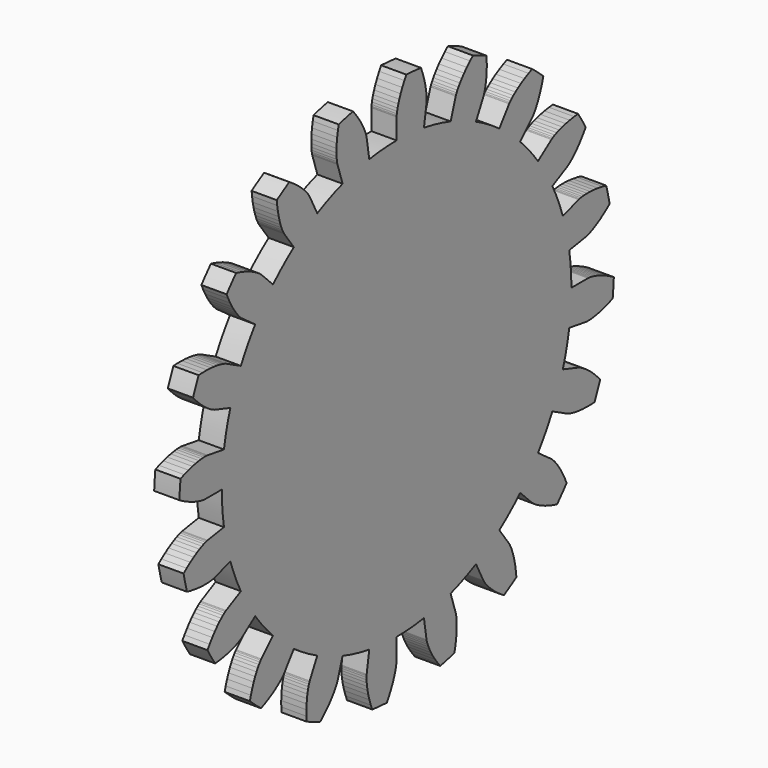
from build123d import *

# Parameters (mm, degrees)
F2_DEPTH = 5.08


# Not quite as in the source:
# - a variable given as a bare number and used for a length is read in inches; the dataset says mm whatever the document's units were


with BuildPart() as f2:
    # F1 (on Right) → F2 (new body)
    with BuildSketch(Plane.YZ):
        with BuildLine():
            ThreePointArc((43.4993825677, -6.8896253625), (43.9058422643, -3.4554647258), (44.0416078431, 0))
            ThreePointArc((44.0416078431, 0), (43.9058422643, 3.4554647258), (43.4993825677, 6.8896253625))
            ThreePointArc((43.4993825677, 6.8896253625), (42.8247347126, 10.2813091677), (41.8860581273, 13.6096052831))
            ThreePointArc((41.8860581273, 13.6096052831), (40.6891400652, 16.8539936563), (39.241359924, 19.994471554))
            ThreePointArc((39.241359924, 19.994471554), (37.5516437498, 23.0116768858), (35.6304092047, 25.8870075774))
            ThreePointArc((35.6304092047, 25.8870075774), (33.4895013385, 28.602736259), (31.1421195602, 31.1421195602))
            ThreePointArc((31.1421195602, 31.1421195602), (28.602736259, 33.4895013385), (25.8870075774, 35.6304092047))
            ThreePointArc((25.8870075774, 35.6304092047), (23.0116768858, 37.5516437498), (19.994471554, 39.241359924))
            ThreePointArc((19.994471554, 39.241359924), (16.8539936563, 40.6891400652), (13.6096052831, 41.8860581273))
            ThreePointArc((13.6096052831, 41.8860581273), (10.2813091677, 42.8247347126), (6.8896253625, 43.4993825677))
            ThreePointArc((6.8896253625, 43.4993825677), (3.4554647258, 43.9058422643), (0, 44.0416078431))
            ThreePointArc((0, 44.0416078431), (-3.4554647258, 43.9058422643), (-6.8896253625, 43.4993825677))
            ThreePointArc((-6.8896253625, 43.4993825677), (-10.2813091677, 42.8247347126), (-13.6096052831, 41.8860581273))
            ThreePointArc((-13.6096052831, 41.8860581273), (-16.8539936563, 40.6891400652), (-19.994471554, 39.241359924))
            ThreePointArc((-19.994471554, 39.241359924), (-23.0116768858, 37.5516437498), (-25.8870075774, 35.6304092047))
            ThreePointArc((-25.8870075774, 35.6304092047), (-28.602736259, 33.4895013385), (-31.1421195602, 31.1421195602))
            ThreePointArc((-31.1421195602, 31.1421195602), (-33.4895013385, 28.602736259), (-35.6304092047, 25.8870075774))
            ThreePointArc((-35.6304092047, 25.8870075774), (-37.5516437498, 23.0116768858), (-39.241359924, 19.994471554))
            ThreePointArc((-39.241359924, 19.994471554), (-40.6891400652, 16.8539936563), (-41.8860581273, 13.6096052831))
            ThreePointArc((-41.8860581273, 13.6096052831), (-42.8247347126, 10.2813091677), (-43.4993825677, 6.8896253625))
            ThreePointArc((-43.4993825677, 6.8896253625), (-43.9058422643, 3.4554647258), (-44.0416078431, 0))
            ThreePointArc((-44.0416078431, 0), (-43.9058422643, -3.4554647258), (-43.4993825677, -6.8896253625))
            ThreePointArc((-43.4993825677, -6.8896253625), (-42.8247347126, -10.2813091677), (-41.8860581273, -13.6096052831))
            ThreePointArc((-41.8860581273, -13.6096052831), (-40.6891400652, -16.8539936563), (-39.241359924, -19.994471554))
            ThreePointArc((-39.241359924, -19.994471554), (-37.5516437498, -23.0116768858), (-35.6304092047, -25.8870075774))
            ThreePointArc((-35.6304092047, -25.8870075774), (-33.4895013385, -28.602736259), (-31.1421195602, -31.1421195602))
            ThreePointArc((-31.1421195602, -31.1421195602), (-28.602736259, -33.4895013385), (-25.8870075774, -35.6304092047))
            ThreePointArc((-25.8870075774, -35.6304092047), (-23.0116768858, -37.5516437498), (-19.994471554, -39.241359924))
            ThreePointArc((-19.994471554, -39.241359924), (-16.8539936563, -40.6891400652), (-13.6096052831, -41.8860581273))
            ThreePointArc((-13.6096052831, -41.8860581273), (-10.2813091677, -42.8247347126), (-6.8896253625, -43.4993825677))
            ThreePointArc((-6.8896253625, -43.4993825677), (-3.4554647258, -43.9058422643), (0, -44.0416078431))
            ThreePointArc((0, -44.0416078431), (3.4554647258, -43.9058422643), (6.8896253625, -43.4993825677))
            ThreePointArc((6.8896253625, -43.4993825677), (10.2813091677, -42.8247347126), (13.6096052831, -41.8860581273))
            ThreePointArc((13.6096052831, -41.8860581273), (16.8539936563, -40.6891400652), (19.994471554, -39.241359924))
            ThreePointArc((19.994471554, -39.241359924), (23.0116768858, -37.5516437498), (25.8870075774, -35.6304092047))
            ThreePointArc((25.8870075774, -35.6304092047), (28.602736259, -33.4895013385), (31.1421195602, -31.1421195602))
            ThreePointArc((31.1421195602, -31.1421195602), (33.4895013385, -28.602736259), (35.6304092047, -25.8870075774))
            ThreePointArc((35.6304092047, -25.8870075774), (37.5516437498, -23.0116768858), (39.241359924, -19.994471554))
            ThreePointArc((39.241359924, -19.994471554), (40.6891400652, -16.8539936563), (41.8860581273, -13.6096052831))
            ThreePointArc((41.8860581273, -13.6096052831), (42.8247347126, -10.2813091677), (43.4993825677, -6.8896253625))
        make_face()
        with BuildLine():
            Line((-45.8576143172, -14.9000421139), (-41.8860581273, -13.6096052831))
            ThreePointArc((-41.8860581273, -13.6096052831), (-42.8247347126, -10.2813091677), (-43.4993825677, -6.8896253625))
            Line((-43.4993825677, -6.8896253625), (-47.6239111058, -7.5428865066))
            Line((-47.6239111058, -7.5428865066), (-47.6830895909, -7.554293021))
            Line((-47.6830895909, -7.554293021), (-47.8589239222, -7.5963654027))
            Line((-47.8589239222, -7.5963654027), (-48.1482035174, -7.6807235949))
            Line((-48.1482035174, -7.6807235949), (-48.5468516924, -7.8187286981))
            Line((-48.5468516924, -7.8187286981), (-49.0499442332, -8.0214256496))
            Line((-49.0499442332, -8.0214256496), (-49.6517315213, -8.2994871485))
            Line((-49.6517315213, -8.2994871485), (-50.345664133, -8.6631590363))
            Line((-50.345664133, -8.6631590363), (-51.1244218199, -9.1222073416))
            Line((-51.1244218199, -9.1222073416), (-51.9799457672, -9.6858671883))
            Line((-51.9799457672, -9.6858671883), (-52.9034740144, -10.3627937613))
            Line((-52.9034740144, -10.3627937613), (-53.6713125986, -10.9868664465))
            ThreePointArc((-53.6713125986, -10.9868664465), (-53.2706187763, -12.7891440512), (-52.8094226758, -14.5768963441))
            Line((-52.8094226758, -14.5768963441), (-51.8419504174, -14.7843577556))
            Line((-51.8419504174, -14.7843577556), (-50.7117624908, -14.9682306981))
            Line((-50.7117624908, -14.9682306981), (-49.6935888566, -15.0820555545))
            Line((-49.6935888566, -15.0820555545), (-48.7913071073, -15.1375219981))
            Line((-48.7913071073, -15.1375219981), (-48.0079050409, -15.1465172096))
            Line((-48.0079050409, -15.1465172096), (-47.3454713621, -15.1210661075))
            Line((-47.3454713621, -15.1210661075), (-46.8051901357, -15.0732711798))
            Line((-46.8051901357, -15.0732711798), (-46.3873390052, -15.0152521429))
            Line((-46.3873390052, -15.0152521429), (-46.0912911807, -14.9590856545))
            Line((-46.0912911807, -14.9590856545), (-45.9155211827, -14.9167453051))
            Line((-45.9155211827, -14.9167453051), (-45.8576143172, -14.9000421139))
        make_face()
        with BuildLine():
            Line((-39.008816688, -28.341564291), (-35.6304092047, -25.8870075774))
            ThreePointArc((-35.6304092047, -25.8870075774), (-37.5516437498, -23.0116768858), (-39.241359924, -19.994471554))
            Line((-39.241359924, -19.994471554), (-42.9621508715, -21.890309234))
            Line((-42.9621508715, -21.890309234), (-43.0149081485, -21.9194446315))
            Line((-43.0149081485, -21.9194446315), (-43.1691354541, -22.0137936409))
            Line((-43.1691354541, -22.0137936409), (-43.4181885832, -22.1834153603))
            Line((-43.4181885832, -22.1834153603), (-43.7546796056, -22.4378550738))
            Line((-43.7546796056, -22.4378550738), (-44.170512242, -22.7860954753))
            Line((-44.170512242, -22.7860954753), (-44.6569202352, -23.2365101747))
            Line((-44.6569202352, -23.2365101747), (-45.2045085737, -23.7968196633))
            Line((-45.2045085737, -23.7968196633), (-45.8032974188, -24.4740499052))
            Line((-45.8032974188, -24.4740499052), (-46.4427685721, -25.2744937142))
            Line((-46.4427685721, -25.2744937142), (-47.1119143146, -26.2036750656))
            Line((-47.1119143146, -26.2036750656), (-47.6493231381, -27.034478631))
            ThreePointArc((-47.6493231381, -27.034478631), (-46.7113062589, -28.6247252905), (-45.720236862, -30.1824613253))
            Line((-45.720236862, -30.1824613253), (-44.7360069646, -30.0808034832))
            Line((-44.7360069646, -30.0808034832), (-43.6043145082, -29.9064297672))
            Line((-43.6043145082, -29.9064297672), (-42.6008000237, -29.7000506824))
            Line((-42.6008000237, -29.7000506824), (-41.7255390128, -29.4739820107))
            Line((-41.7255390128, -29.4739820107), (-40.9776996994, -29.2404524133))
            Line((-40.9776996994, -29.2404524133), (-40.3555526557, -29.0115437125))
            Line((-40.3555526557, -29.0115437125), (-39.8564841196, -28.7991319543))
            Line((-39.8564841196, -28.7991319543), (-39.4770129475, -28.6148294707))
            Line((-39.4770129475, -28.6148294707), (-39.2128111343, -28.469928157))
            Line((-39.2128111343, -28.469928157), (-39.0587278198, -28.3753441754))
            Line((-39.0587278198, -28.3753441754), (-39.008816688, -28.341564291))
        make_face()
        with BuildLine():
            Line((-28.341564291, -39.008816688), (-25.8870075774, -35.6304092047))
            ThreePointArc((-25.8870075774, -35.6304092047), (-28.602736259, -33.4895013385), (-31.1421195602, -31.1421195602))
            Line((-31.1421195602, -31.1421195602), (-34.0949559749, -34.0949559749))
            Line((-34.0949559749, -34.0949559749), (-34.1361277941, -34.1389682797))
            Line((-34.1361277941, -34.1389682797), (-34.2536512308, -34.2763583784))
            Line((-34.2536512308, -34.2763583784), (-34.4380988382, -34.5146398693))
            Line((-34.4380988382, -34.5146398693), (-34.6794946222, -34.8606078612))
            Line((-34.6794946222, -34.8606078612), (-34.9673627586, -35.3203035157))
            Line((-34.9673627586, -35.3203035157), (-35.2907784534, -35.8989816867))
            Line((-35.2907784534, -35.8989816867), (-35.6384207569, -36.6010817796))
            Line((-35.6384207569, -36.6010817796), (-35.9986271361, -37.4302019433))
            Line((-35.9986271361, -37.4302019433), (-36.3594496034, -38.3890766975))
            Line((-36.3594496034, -38.3890766975), (-36.7087121936, -39.4795580828))
            Line((-36.7087121936, -39.4795580828), (-36.9630859365, -40.4357676868))
            ThreePointArc((-36.9630859365, -40.4357676868), (-35.5795656281, -41.6583189782), (-34.1556357126, -42.8335566985))
            Line((-34.1556357126, -42.8335566985), (-33.2509914559, -42.4327305806))
            Line((-33.2509914559, -42.4327305806), (-32.2285724125, -41.9171791203))
            Line((-32.2285724125, -41.9171791203), (-31.3379480673, -41.4107979171))
            Line((-31.3379480673, -41.4107979171), (-30.5753844409, -40.9253233069))
            Line((-30.5753844409, -40.9253233069), (-29.936311603, -40.4721284046))
            Line((-29.936311603, -40.4721284046), (-29.4153512817, -40.0621692835))
            Line((-29.4153512817, -40.0621692835), (-29.0063477414, -39.7059330378))
            Line((-29.0063477414, -39.7059330378), (-28.70240181, -39.4133879188))
            Line((-28.70240181, -39.4133879188), (-28.4959079224, -39.1939357299))
            Line((-28.4959079224, -39.1939357299), (-28.3785940398, -39.0563666551))
            Line((-28.3785940398, -39.0563666551), (-28.341564291, -39.008816688))
        make_face()
        with BuildLine():
            Line((-14.9000421139, -45.8576143172), (-13.6096052831, -41.8860581273))
            ThreePointArc((-13.6096052831, -41.8860581273), (-16.8539936563, -40.6891400652), (-19.994471554, -39.241359924))
            Line((-19.994471554, -39.241359924), (-21.890309234, -42.9621508715))
            Line((-21.890309234, -42.9621508715), (-21.9158654108, -43.0167318526))
            Line((-21.9158654108, -43.0167318526), (-21.9851809658, -43.1837143403))
            Line((-21.9851809658, -43.1837143403), (-22.0869680345, -43.4673309502))
            Line((-22.0869680345, -43.4673309502), (-22.2096390789, -43.8709614629))
            Line((-22.2096390789, -43.8709614629), (-22.3413641764, -44.397114157))
            Line((-22.3413641764, -44.397114157), (-22.4701293913, -45.0474107484))
            Line((-22.4701293913, -45.0474107484), (-22.5837960089, -45.8225749965))
            Line((-22.5837960089, -45.8225749965), (-22.6701604121, -46.7224250236))
            Line((-22.6701604121, -46.7224250236), (-22.7170143763, -47.7458693813))
            Line((-22.7170143763, -47.7458693813), (-22.7122055586, -48.8909068846))
            Line((-22.7122055586, -48.8909068846), (-22.6586443465, -49.8789220689))
            ThreePointArc((-22.6586443465, -49.8789220689), (-20.9650492162, -50.6141061537), (-19.2476429633, -51.2918051031))
            Line((-19.2476429633, -51.2918051031), (-18.5111372303, -50.6310463626))
            Line((-18.5111372303, -50.6310463626), (-17.6980730994, -49.824782927))
            Line((-17.6980730994, -49.824782927), (-17.0075194097, -49.0679677257))
            Line((-17.0075194097, -49.0679677257), (-16.4322982086, -48.3706088143))
            Line((-16.4322982086, -48.3706088143), (-15.9645487484, -47.7421104818))
            Line((-15.9645487484, -47.7421104818), (-15.5957703755, -47.1912305956))
            Line((-15.5957703755, -47.1912305956), (-15.3168679472, -46.726040748))
            Line((-15.3168679472, -46.726040748), (-15.1181996019, -46.3538893481))
            Line((-15.1181996019, -46.3538893481), (-14.9896267004, -46.0813677933))
            Line((-14.9896267004, -46.0813677933), (-14.9205657499, -45.914279845))
            Line((-14.9205657499, -45.914279845), (-14.9000421139, -45.8576143172))
        make_face()
        with BuildLine():
            Line((0, -48.2175491482), (0, -44.0416078431))
            ThreePointArc((0, -44.0416078431), (-3.4554647258, -43.9058422643), (-6.8896253625, -43.4993825677))
            Line((-6.8896253625, -43.4993825677), (-7.5428865066, -47.6239111058))
            Line((-7.5428865066, -47.6239111058), (-7.5503254243, -47.6837179965))
            Line((-7.5503254243, -47.6837179965), (-7.564648008, -47.863947464))
            Line((-7.564648008, -47.863947464), (-7.5738109107, -48.1651368231))
            Line((-7.5738109107, -48.1651368231), (-7.5657493189, -48.5869196898))
            Line((-7.5657493189, -48.5869196898), (-7.5284372071, -49.1280259317))
            Line((-7.5284372071, -49.1280259317), (-7.4499475057, -49.7862853821))
            Line((-7.4499475057, -49.7862853821), (-7.318511957, -50.5586353081))
            Line((-7.318511957, -50.5586353081), (-7.1225804347, -51.4411316084))
            Line((-7.1225804347, -51.4411316084), (-6.8508795033, -52.428963705))
            Line((-6.8508795033, -52.428963705), (-6.4924699982, -53.5164730775))
            Line((-6.4924699982, -53.5164730775), (-6.1362167757, -54.4395800319))
            ThreePointArc((-6.1362167757, -54.4395800319), (-4.298327715, -54.6154319696), (-2.4555568145, -54.7292542531))
            Line((-2.4555568145, -54.7292542531), (-1.9592839178, -53.8732425593))
            Line((-1.9592839178, -53.8732425593), (-1.4351630815, -52.8551898311))
            Line((-1.4351630815, -52.8551898311), (-1.0122762539, -51.9220229766))
            Line((-1.0122762539, -51.9220229766), (-0.6807041371, -51.0810421131))
            Line((-0.6807041371, -51.0810421131), (-0.4300646306, -50.3387621461))
            Line((-0.4300646306, -50.3387621461), (-0.2495668027, -49.7008854563))
            Line((-0.2495668027, -49.7008854563), (-0.1280663995, -49.1722780304))
            Line((-0.1280663995, -49.1722780304), (-0.0541226821, -48.7569491214))
            Line((-0.0541226821, -48.7569491214), (-0.016056378, -48.4580345094))
            Line((-0.016056378, -48.4580345094), (-0.0020085267, -48.27778342))
            Line((-0.0020085267, -48.27778342), (0, -48.2175491482))
        make_face()
        with BuildLine():
            Line((14.9000421139, -45.8576143172), (13.6096052831, -41.8860581273))
            ThreePointArc((13.6096052831, -41.8860581273), (10.2813091677, -42.8247347126), (6.8896253625, -43.4993825677))
            Line((6.8896253625, -43.4993825677), (7.5428865066, -47.6239111058))
            Line((7.5428865066, -47.6239111058), (7.554293021, -47.6830895909))
            Line((7.554293021, -47.6830895909), (7.5963654027, -47.8589239222))
            Line((7.5963654027, -47.8589239222), (7.6807235949, -48.1482035174))
            Line((7.6807235949, -48.1482035174), (7.8187286981, -48.5468516924))
            Line((7.8187286981, -48.5468516924), (8.0214256496, -49.0499442332))
            Line((8.0214256496, -49.0499442332), (8.2994871485, -49.6517315213))
            Line((8.2994871485, -49.6517315213), (8.6631590363, -50.345664133))
            Line((8.6631590363, -50.345664133), (9.1222073416, -51.1244218199))
            Line((9.1222073416, -51.1244218199), (9.6858671883, -51.9799457672))
            Line((9.6858671883, -51.9799457672), (10.3627937613, -52.9034740144))
            Line((10.3627937613, -52.9034740144), (10.9868664465, -53.6713125986))
            ThreePointArc((10.9868664465, -53.6713125986), (12.7891440512, -53.2706187763), (14.5768963441, -52.8094226758))
            Line((14.5768963441, -52.8094226758), (14.7843577556, -51.8419504174))
            Line((14.7843577556, -51.8419504174), (14.9682306981, -50.7117624908))
            Line((14.9682306981, -50.7117624908), (15.0820555545, -49.6935888566))
            Line((15.0820555545, -49.6935888566), (15.1375219981, -48.7913071073))
            Line((15.1375219981, -48.7913071073), (15.1465172096, -48.0079050409))
            Line((15.1465172096, -48.0079050409), (15.1210661075, -47.3454713621))
            Line((15.1210661075, -47.3454713621), (15.0732711798, -46.8051901357))
            Line((15.0732711798, -46.8051901357), (15.0152521429, -46.3873390052))
            Line((15.0152521429, -46.3873390052), (14.9590856545, -46.0912911807))
            Line((14.9590856545, -46.0912911807), (14.9167453051, -45.9155211827))
            Line((14.9167453051, -45.9155211827), (14.9000421139, -45.8576143172))
        make_face()
        with BuildLine():
            Line((28.341564291, -39.008816688), (25.8870075774, -35.6304092047))
            ThreePointArc((25.8870075774, -35.6304092047), (23.0116768858, -37.5516437498), (19.994471554, -39.241359924))
            Line((19.994471554, -39.241359924), (21.890309234, -42.9621508715))
            Line((21.890309234, -42.9621508715), (21.9194446315, -43.0149081485))
            Line((21.9194446315, -43.0149081485), (22.0137936409, -43.1691354541))
            Line((22.0137936409, -43.1691354541), (22.1834153603, -43.4181885832))
            Line((22.1834153603, -43.4181885832), (22.4378550738, -43.7546796056))
            Line((22.4378550738, -43.7546796056), (22.7860954753, -44.170512242))
            Line((22.7860954753, -44.170512242), (23.2365101747, -44.6569202352))
            Line((23.2365101747, -44.6569202352), (23.7968196633, -45.2045085737))
            Line((23.7968196633, -45.2045085737), (24.4740499052, -45.8032974188))
            Line((24.4740499052, -45.8032974188), (25.2744937142, -46.4427685721))
            Line((25.2744937142, -46.4427685721), (26.2036750656, -47.1119143146))
            Line((26.2036750656, -47.1119143146), (27.034478631, -47.6493231381))
            ThreePointArc((27.034478631, -47.6493231381), (28.6247252905, -46.7113062589), (30.1824613253, -45.720236862))
            Line((30.1824613253, -45.720236862), (30.0808034832, -44.7360069646))
            Line((30.0808034832, -44.7360069646), (29.9064297672, -43.6043145082))
            Line((29.9064297672, -43.6043145082), (29.7000506824, -42.6008000237))
            Line((29.7000506824, -42.6008000237), (29.4739820107, -41.7255390128))
            Line((29.4739820107, -41.7255390128), (29.2404524133, -40.9776996994))
            Line((29.2404524133, -40.9776996994), (29.0115437125, -40.3555526557))
            Line((29.0115437125, -40.3555526557), (28.7991319543, -39.8564841196))
            Line((28.7991319543, -39.8564841196), (28.6148294707, -39.4770129475))
            Line((28.6148294707, -39.4770129475), (28.469928157, -39.2128111343))
            Line((28.469928157, -39.2128111343), (28.3753441754, -39.0587278198))
            Line((28.3753441754, -39.0587278198), (28.341564291, -39.008816688))
        make_face()
        with BuildLine():
            Line((39.008816688, -28.341564291), (35.6304092047, -25.8870075774))
            ThreePointArc((35.6304092047, -25.8870075774), (33.4895013385, -28.602736259), (31.1421195602, -31.1421195602))
            Line((31.1421195602, -31.1421195602), (34.0949559749, -34.0949559749))
            Line((34.0949559749, -34.0949559749), (34.1389682797, -34.1361277941))
            Line((34.1389682797, -34.1361277941), (34.2763583784, -34.2536512308))
            Line((34.2763583784, -34.2536512308), (34.5146398693, -34.4380988382))
            Line((34.5146398693, -34.4380988382), (34.8606078612, -34.6794946222))
            Line((34.8606078612, -34.6794946222), (35.3203035157, -34.9673627586))
            Line((35.3203035157, -34.9673627586), (35.8989816867, -35.2907784534))
            Line((35.8989816867, -35.2907784534), (36.6010817796, -35.6384207569))
            Line((36.6010817796, -35.6384207569), (37.4302019433, -35.9986271361))
            Line((37.4302019433, -35.9986271361), (38.3890766975, -36.3594496034))
            Line((38.3890766975, -36.3594496034), (39.4795580828, -36.7087121936))
            Line((39.4795580828, -36.7087121936), (40.4357676868, -36.9630859365))
            ThreePointArc((40.4357676868, -36.9630859365), (41.6583189782, -35.5795656281), (42.8335566985, -34.1556357126))
            Line((42.8335566985, -34.1556357126), (42.4327305806, -33.2509914559))
            Line((42.4327305806, -33.2509914559), (41.9171791203, -32.2285724125))
            Line((41.9171791203, -32.2285724125), (41.4107979171, -31.3379480673))
            Line((41.4107979171, -31.3379480673), (40.9253233069, -30.5753844409))
            Line((40.9253233069, -30.5753844409), (40.4721284046, -29.936311603))
            Line((40.4721284046, -29.936311603), (40.0621692835, -29.4153512817))
            Line((40.0621692835, -29.4153512817), (39.7059330378, -29.0063477414))
            Line((39.7059330378, -29.0063477414), (39.4133879188, -28.70240181))
            Line((39.4133879188, -28.70240181), (39.1939357299, -28.4959079224))
            Line((39.1939357299, -28.4959079224), (39.0563666551, -28.3785940398))
            Line((39.0563666551, -28.3785940398), (39.008816688, -28.341564291))
        make_face()
        with BuildLine():
            Line((45.8576143172, -14.9000421139), (41.8860581273, -13.6096052831))
            ThreePointArc((41.8860581273, -13.6096052831), (40.6891400652, -16.8539936563), (39.241359924, -19.994471554))
            Line((39.241359924, -19.994471554), (42.9621508715, -21.890309234))
            Line((42.9621508715, -21.890309234), (43.0167318526, -21.9158654108))
            Line((43.0167318526, -21.9158654108), (43.1837143403, -21.9851809658))
            Line((43.1837143403, -21.9851809658), (43.4673309502, -22.0869680345))
            Line((43.4673309502, -22.0869680345), (43.8709614629, -22.2096390789))
            Line((43.8709614629, -22.2096390789), (44.397114157, -22.3413641764))
            Line((44.397114157, -22.3413641764), (45.0474107484, -22.4701293913))
            Line((45.0474107484, -22.4701293913), (45.8225749965, -22.5837960089))
            Line((45.8225749965, -22.5837960089), (46.7224250236, -22.6701604121))
            Line((46.7224250236, -22.6701604121), (47.7458693813, -22.7170143763))
            Line((47.7458693813, -22.7170143763), (48.8909068846, -22.7122055586))
            Line((48.8909068846, -22.7122055586), (49.8789220689, -22.6586443465))
            ThreePointArc((49.8789220689, -22.6586443465), (50.6141061537, -20.9650492162), (51.2918051031, -19.2476429633))
            Line((51.2918051031, -19.2476429633), (50.6310463626, -18.5111372303))
            Line((50.6310463626, -18.5111372303), (49.824782927, -17.6980730994))
            Line((49.824782927, -17.6980730994), (49.0679677257, -17.0075194097))
            Line((49.0679677257, -17.0075194097), (48.3706088143, -16.4322982086))
            Line((48.3706088143, -16.4322982086), (47.7421104818, -15.9645487484))
            Line((47.7421104818, -15.9645487484), (47.1912305956, -15.5957703755))
            Line((47.1912305956, -15.5957703755), (46.726040748, -15.3168679472))
            Line((46.726040748, -15.3168679472), (46.3538893481, -15.1181996019))
            Line((46.3538893481, -15.1181996019), (46.0813677933, -14.9896267004))
            Line((46.0813677933, -14.9896267004), (45.914279845, -14.9205657499))
            Line((45.914279845, -14.9205657499), (45.8576143172, -14.9000421139))
        make_face()
        with BuildLine():
            Line((48.2175491482, 0), (44.0416078431, 0))
            ThreePointArc((44.0416078431, 0), (43.9058422643, -3.4554647258), (43.4993825677, -6.8896253625))
            Line((43.4993825677, -6.8896253625), (47.6239111058, -7.5428865066))
            Line((47.6239111058, -7.5428865066), (47.6837179965, -7.5503254243))
            Line((47.6837179965, -7.5503254243), (47.863947464, -7.564648008))
            Line((47.863947464, -7.564648008), (48.1651368231, -7.5738109107))
            Line((48.1651368231, -7.5738109107), (48.5869196898, -7.5657493189))
            Line((48.5869196898, -7.5657493189), (49.1280259317, -7.5284372071))
            Line((49.1280259317, -7.5284372071), (49.7862853821, -7.4499475057))
            Line((49.7862853821, -7.4499475057), (50.5586353081, -7.318511957))
            Line((50.5586353081, -7.318511957), (51.4411316084, -7.1225804347))
            Line((51.4411316084, -7.1225804347), (52.428963705, -6.8508795033))
            Line((52.428963705, -6.8508795033), (53.5164730775, -6.4924699982))
            Line((53.5164730775, -6.4924699982), (54.4395800319, -6.1362167757))
            ThreePointArc((54.4395800319, -6.1362167757), (54.6154319696, -4.298327715), (54.7292542531, -2.4555568145))
            Line((54.7292542531, -2.4555568145), (53.8732425593, -1.9592839178))
            Line((53.8732425593, -1.9592839178), (52.8551898311, -1.4351630815))
            Line((52.8551898311, -1.4351630815), (51.9220229766, -1.0122762539))
            Line((51.9220229766, -1.0122762539), (51.0810421131, -0.6807041371))
            Line((51.0810421131, -0.6807041371), (50.3387621461, -0.4300646306))
            Line((50.3387621461, -0.4300646306), (49.7008854563, -0.2495668027))
            Line((49.7008854563, -0.2495668027), (49.1722780304, -0.1280663995))
            Line((49.1722780304, -0.1280663995), (48.7569491214, -0.0541226821))
            Line((48.7569491214, -0.0541226821), (48.4580345094, -0.016056378))
            Line((48.4580345094, -0.016056378), (48.27778342, -0.0020085267))
            Line((48.27778342, -0.0020085267), (48.2175491482, 0))
        make_face()
        with BuildLine():
            ThreePointArc((41.8860581273, 13.6096052831), (42.8247347126, 10.2813091677), (43.4993825677, 6.8896253625))
            Line((43.4993825677, 6.8896253625), (47.6239111058, 7.5428865066))
            Line((47.6239111058, 7.5428865066), (47.6830895909, 7.554293021))
            Line((47.6830895909, 7.554293021), (47.8589239222, 7.5963654027))
            Line((47.8589239222, 7.5963654027), (48.1482035174, 7.6807235949))
            Line((48.1482035174, 7.6807235949), (48.5468516924, 7.8187286981))
            Line((48.5468516924, 7.8187286981), (49.0499442332, 8.0214256496))
            Line((49.0499442332, 8.0214256496), (49.6517315213, 8.2994871485))
            Line((49.6517315213, 8.2994871485), (50.345664133, 8.6631590363))
            Line((50.345664133, 8.6631590363), (51.1244218199, 9.1222073416))
            Line((51.1244218199, 9.1222073416), (51.9799457672, 9.6858671883))
            Line((51.9799457672, 9.6858671883), (52.9034740144, 10.3627937613))
            Line((52.9034740144, 10.3627937613), (53.6713125986, 10.9868664465))
            ThreePointArc((53.6713125986, 10.9868664465), (53.2706187763, 12.7891440512), (52.8094226758, 14.5768963441))
            Line((52.8094226758, 14.5768963441), (51.8419504174, 14.7843577556))
            Line((51.8419504174, 14.7843577556), (50.7117624908, 14.9682306981))
            Line((50.7117624908, 14.9682306981), (49.6935888566, 15.0820555545))
            Line((49.6935888566, 15.0820555545), (48.7913071073, 15.1375219981))
            Line((48.7913071073, 15.1375219981), (48.0079050409, 15.1465172096))
            Line((48.0079050409, 15.1465172096), (47.3454713621, 15.1210661075))
            Line((47.3454713621, 15.1210661075), (46.8051901357, 15.0732711798))
            Line((46.8051901357, 15.0732711798), (46.3873390052, 15.0152521429))
            Line((46.3873390052, 15.0152521429), (46.0912911807, 14.9590856545))
            Line((46.0912911807, 14.9590856545), (45.9155211827, 14.9167453051))
            Line((45.9155211827, 14.9167453051), (45.8576143172, 14.9000421139))
            Line((45.8576143172, 14.9000421139), (41.8860581273, 13.6096052831))
        make_face()
        with BuildLine():
            ThreePointArc((35.6304092047, 25.8870075774), (37.5516437498, 23.0116768858), (39.241359924, 19.994471554))
            Line((39.241359924, 19.994471554), (42.9621508715, 21.890309234))
            Line((42.9621508715, 21.890309234), (43.0149081485, 21.9194446315))
            Line((43.0149081485, 21.9194446315), (43.1691354541, 22.0137936409))
            Line((43.1691354541, 22.0137936409), (43.4181885832, 22.1834153603))
            Line((43.4181885832, 22.1834153603), (43.7546796056, 22.4378550738))
            Line((43.7546796056, 22.4378550738), (44.170512242, 22.7860954753))
            Line((44.170512242, 22.7860954753), (44.6569202352, 23.2365101747))
            Line((44.6569202352, 23.2365101747), (45.2045085737, 23.7968196633))
            Line((45.2045085737, 23.7968196633), (45.8032974188, 24.4740499052))
            Line((45.8032974188, 24.4740499052), (46.4427685721, 25.2744937142))
            Line((46.4427685721, 25.2744937142), (47.1119143146, 26.2036750656))
            Line((47.1119143146, 26.2036750656), (47.6493231381, 27.034478631))
            ThreePointArc((47.6493231381, 27.034478631), (46.7113062589, 28.6247252905), (45.720236862, 30.1824613253))
            Line((45.720236862, 30.1824613253), (44.7360069646, 30.0808034832))
            Line((44.7360069646, 30.0808034832), (43.6043145082, 29.9064297672))
            Line((43.6043145082, 29.9064297672), (42.6008000237, 29.7000506824))
            Line((42.6008000237, 29.7000506824), (41.7255390128, 29.4739820107))
            Line((41.7255390128, 29.4739820107), (40.9776996994, 29.2404524133))
            Line((40.9776996994, 29.2404524133), (40.3555526557, 29.0115437125))
            Line((40.3555526557, 29.0115437125), (39.8564841196, 28.7991319543))
            Line((39.8564841196, 28.7991319543), (39.4770129475, 28.6148294707))
            Line((39.4770129475, 28.6148294707), (39.2128111343, 28.469928157))
            Line((39.2128111343, 28.469928157), (39.0587278198, 28.3753441754))
            Line((39.0587278198, 28.3753441754), (39.008816688, 28.341564291))
            Line((39.008816688, 28.341564291), (35.6304092047, 25.8870075774))
        make_face()
        with BuildLine():
            ThreePointArc((25.8870075774, 35.6304092047), (28.602736259, 33.4895013385), (31.1421195602, 31.1421195602))
            Line((31.1421195602, 31.1421195602), (34.0949559749, 34.0949559749))
            Line((34.0949559749, 34.0949559749), (34.1361277941, 34.1389682797))
            Line((34.1361277941, 34.1389682797), (34.2536512308, 34.2763583784))
            Line((34.2536512308, 34.2763583784), (34.4380988382, 34.5146398693))
            Line((34.4380988382, 34.5146398693), (34.6794946222, 34.8606078612))
            Line((34.6794946222, 34.8606078612), (34.9673627586, 35.3203035157))
            Line((34.9673627586, 35.3203035157), (35.2907784534, 35.8989816867))
            Line((35.2907784534, 35.8989816867), (35.6384207569, 36.6010817796))
            Line((35.6384207569, 36.6010817796), (35.9986271361, 37.4302019433))
            Line((35.9986271361, 37.4302019433), (36.3594496034, 38.3890766975))
            Line((36.3594496034, 38.3890766975), (36.7087121936, 39.4795580828))
            Line((36.7087121936, 39.4795580828), (36.9630859365, 40.4357676868))
            ThreePointArc((36.9630859365, 40.4357676868), (35.5795656281, 41.6583189782), (34.1556357126, 42.8335566985))
            Line((34.1556357126, 42.8335566985), (33.2509914559, 42.4327305806))
            Line((33.2509914559, 42.4327305806), (32.2285724125, 41.9171791203))
            Line((32.2285724125, 41.9171791203), (31.3379480673, 41.4107979171))
            Line((31.3379480673, 41.4107979171), (30.5753844409, 40.9253233069))
            Line((30.5753844409, 40.9253233069), (29.936311603, 40.4721284046))
            Line((29.936311603, 40.4721284046), (29.4153512817, 40.0621692835))
            Line((29.4153512817, 40.0621692835), (29.0063477414, 39.7059330378))
            Line((29.0063477414, 39.7059330378), (28.70240181, 39.4133879188))
            Line((28.70240181, 39.4133879188), (28.4959079224, 39.1939357299))
            Line((28.4959079224, 39.1939357299), (28.3785940398, 39.0563666551))
            Line((28.3785940398, 39.0563666551), (28.341564291, 39.008816688))
            Line((28.341564291, 39.008816688), (25.8870075774, 35.6304092047))
        make_face()
        with BuildLine():
            ThreePointArc((13.6096052831, 41.8860581273), (16.8539936563, 40.6891400652), (19.994471554, 39.241359924))
            Line((19.994471554, 39.241359924), (21.890309234, 42.9621508715))
            Line((21.890309234, 42.9621508715), (21.9158654108, 43.0167318526))
            Line((21.9158654108, 43.0167318526), (21.9851809658, 43.1837143403))
            Line((21.9851809658, 43.1837143403), (22.0869680345, 43.4673309502))
            Line((22.0869680345, 43.4673309502), (22.2096390789, 43.8709614629))
            Line((22.2096390789, 43.8709614629), (22.3413641764, 44.397114157))
            Line((22.3413641764, 44.397114157), (22.4701293913, 45.0474107484))
            Line((22.4701293913, 45.0474107484), (22.5837960089, 45.8225749965))
            Line((22.5837960089, 45.8225749965), (22.6701604121, 46.7224250236))
            Line((22.6701604121, 46.7224250236), (22.7170143763, 47.7458693813))
            Line((22.7170143763, 47.7458693813), (22.7122055586, 48.8909068846))
            Line((22.7122055586, 48.8909068846), (22.6586443465, 49.8789220689))
            ThreePointArc((22.6586443465, 49.8789220689), (20.9650492162, 50.6141061537), (19.2476429633, 51.2918051031))
            Line((19.2476429633, 51.2918051031), (18.5111372303, 50.6310463626))
            Line((18.5111372303, 50.6310463626), (17.6980730994, 49.824782927))
            Line((17.6980730994, 49.824782927), (17.0075194097, 49.0679677257))
            Line((17.0075194097, 49.0679677257), (16.4322982086, 48.3706088143))
            Line((16.4322982086, 48.3706088143), (15.9645487484, 47.7421104818))
            Line((15.9645487484, 47.7421104818), (15.5957703755, 47.1912305956))
            Line((15.5957703755, 47.1912305956), (15.3168679472, 46.726040748))
            Line((15.3168679472, 46.726040748), (15.1181996019, 46.3538893481))
            Line((15.1181996019, 46.3538893481), (14.9896267004, 46.0813677933))
            Line((14.9896267004, 46.0813677933), (14.9205657499, 45.914279845))
            Line((14.9205657499, 45.914279845), (14.9000421139, 45.8576143172))
            Line((14.9000421139, 45.8576143172), (13.6096052831, 41.8860581273))
        make_face()
        with BuildLine():
            ThreePointArc((0, 44.0416078431), (3.4554647258, 43.9058422643), (6.8896253625, 43.4993825677))
            Line((6.8896253625, 43.4993825677), (7.5428865066, 47.6239111058))
            Line((7.5428865066, 47.6239111058), (7.5503254243, 47.6837179965))
            Line((7.5503254243, 47.6837179965), (7.564648008, 47.863947464))
            Line((7.564648008, 47.863947464), (7.5738109107, 48.1651368231))
            Line((7.5738109107, 48.1651368231), (7.5657493189, 48.5869196898))
            Line((7.5657493189, 48.5869196898), (7.5284372071, 49.1280259317))
            Line((7.5284372071, 49.1280259317), (7.4499475057, 49.7862853821))
            Line((7.4499475057, 49.7862853821), (7.318511957, 50.5586353081))
            Line((7.318511957, 50.5586353081), (7.1225804347, 51.4411316084))
            Line((7.1225804347, 51.4411316084), (6.8508795033, 52.428963705))
            Line((6.8508795033, 52.428963705), (6.4924699982, 53.5164730775))
            Line((6.4924699982, 53.5164730775), (6.1362167757, 54.4395800319))
            ThreePointArc((6.1362167757, 54.4395800319), (4.298327715, 54.6154319696), (2.4555568145, 54.7292542531))
            Line((2.4555568145, 54.7292542531), (1.9592839178, 53.8732425593))
            Line((1.9592839178, 53.8732425593), (1.4351630815, 52.8551898311))
            Line((1.4351630815, 52.8551898311), (1.0122762539, 51.9220229766))
            Line((1.0122762539, 51.9220229766), (0.6807041371, 51.0810421131))
            Line((0.6807041371, 51.0810421131), (0.4300646306, 50.3387621461))
            Line((0.4300646306, 50.3387621461), (0.2495668027, 49.7008854563))
            Line((0.2495668027, 49.7008854563), (0.1280663995, 49.1722780304))
            Line((0.1280663995, 49.1722780304), (0.0541226821, 48.7569491214))
            Line((0.0541226821, 48.7569491214), (0.016056378, 48.4580345094))
            Line((0.016056378, 48.4580345094), (0.0020085267, 48.27778342))
            Line((0.0020085267, 48.27778342), (0, 48.2175491482))
            Line((0, 48.2175491482), (0, 44.0416078431))
        make_face()
        with BuildLine():
            ThreePointArc((-13.6096052831, 41.8860581273), (-10.2813091677, 42.8247347126), (-6.8896253625, 43.4993825677))
            Line((-6.8896253625, 43.4993825677), (-7.5428865066, 47.6239111058))
            Line((-7.5428865066, 47.6239111058), (-7.554293021, 47.6830895909))
            Line((-7.554293021, 47.6830895909), (-7.5963654027, 47.8589239222))
            Line((-7.5963654027, 47.8589239222), (-7.6807235949, 48.1482035174))
            Line((-7.6807235949, 48.1482035174), (-7.8187286981, 48.5468516924))
            Line((-7.8187286981, 48.5468516924), (-8.0214256496, 49.0499442332))
            Line((-8.0214256496, 49.0499442332), (-8.2994871485, 49.6517315213))
            Line((-8.2994871485, 49.6517315213), (-8.6631590363, 50.345664133))
            Line((-8.6631590363, 50.345664133), (-9.1222073416, 51.1244218199))
            Line((-9.1222073416, 51.1244218199), (-9.6858671883, 51.9799457672))
            Line((-9.6858671883, 51.9799457672), (-10.3627937613, 52.9034740144))
            Line((-10.3627937613, 52.9034740144), (-10.9868664465, 53.6713125986))
            ThreePointArc((-10.9868664465, 53.6713125986), (-12.7891440512, 53.2706187763), (-14.5768963441, 52.8094226758))
            Line((-14.5768963441, 52.8094226758), (-14.7843577556, 51.8419504174))
            Line((-14.7843577556, 51.8419504174), (-14.9682306981, 50.7117624908))
            Line((-14.9682306981, 50.7117624908), (-15.0820555545, 49.6935888566))
            Line((-15.0820555545, 49.6935888566), (-15.1375219981, 48.7913071073))
            Line((-15.1375219981, 48.7913071073), (-15.1465172096, 48.0079050409))
            Line((-15.1465172096, 48.0079050409), (-15.1210661075, 47.3454713621))
            Line((-15.1210661075, 47.3454713621), (-15.0732711798, 46.8051901357))
            Line((-15.0732711798, 46.8051901357), (-15.0152521429, 46.3873390052))
            Line((-15.0152521429, 46.3873390052), (-14.9590856545, 46.0912911807))
            Line((-14.9590856545, 46.0912911807), (-14.9167453051, 45.9155211827))
            Line((-14.9167453051, 45.9155211827), (-14.9000421139, 45.8576143172))
            Line((-14.9000421139, 45.8576143172), (-13.6096052831, 41.8860581273))
        make_face()
        with BuildLine():
            ThreePointArc((-25.8870075774, 35.6304092047), (-23.0116768858, 37.5516437498), (-19.994471554, 39.241359924))
            Line((-19.994471554, 39.241359924), (-21.890309234, 42.9621508715))
            Line((-21.890309234, 42.9621508715), (-21.9194446315, 43.0149081485))
            Line((-21.9194446315, 43.0149081485), (-22.0137936409, 43.1691354541))
            Line((-22.0137936409, 43.1691354541), (-22.1834153603, 43.4181885832))
            Line((-22.1834153603, 43.4181885832), (-22.4378550738, 43.7546796056))
            Line((-22.4378550738, 43.7546796056), (-22.7860954753, 44.170512242))
            Line((-22.7860954753, 44.170512242), (-23.2365101747, 44.6569202352))
            Line((-23.2365101747, 44.6569202352), (-23.7968196633, 45.2045085737))
            Line((-23.7968196633, 45.2045085737), (-24.4740499052, 45.8032974188))
            Line((-24.4740499052, 45.8032974188), (-25.2744937142, 46.4427685721))
            Line((-25.2744937142, 46.4427685721), (-26.2036750656, 47.1119143146))
            Line((-26.2036750656, 47.1119143146), (-27.034478631, 47.6493231381))
            ThreePointArc((-27.034478631, 47.6493231381), (-28.6247252905, 46.7113062589), (-30.1824613253, 45.720236862))
            Line((-30.1824613253, 45.720236862), (-30.0808034832, 44.7360069646))
            Line((-30.0808034832, 44.7360069646), (-29.9064297672, 43.6043145082))
            Line((-29.9064297672, 43.6043145082), (-29.7000506824, 42.6008000237))
            Line((-29.7000506824, 42.6008000237), (-29.4739820107, 41.7255390128))
            Line((-29.4739820107, 41.7255390128), (-29.2404524133, 40.9776996994))
            Line((-29.2404524133, 40.9776996994), (-29.0115437125, 40.3555526557))
            Line((-29.0115437125, 40.3555526557), (-28.7991319543, 39.8564841196))
            Line((-28.7991319543, 39.8564841196), (-28.6148294707, 39.4770129475))
            Line((-28.6148294707, 39.4770129475), (-28.469928157, 39.2128111343))
            Line((-28.469928157, 39.2128111343), (-28.3753441754, 39.0587278198))
            Line((-28.3753441754, 39.0587278198), (-28.341564291, 39.008816688))
            Line((-28.341564291, 39.008816688), (-25.8870075774, 35.6304092047))
        make_face()
        with BuildLine():
            ThreePointArc((-35.6304092047, 25.8870075774), (-33.4895013385, 28.602736259), (-31.1421195602, 31.1421195602))
            Line((-31.1421195602, 31.1421195602), (-34.0949559749, 34.0949559749))
            Line((-34.0949559749, 34.0949559749), (-34.1389682797, 34.1361277941))
            Line((-34.1389682797, 34.1361277941), (-34.2763583784, 34.2536512308))
            Line((-34.2763583784, 34.2536512308), (-34.5146398693, 34.4380988382))
            Line((-34.5146398693, 34.4380988382), (-34.8606078612, 34.6794946222))
            Line((-34.8606078612, 34.6794946222), (-35.3203035157, 34.9673627586))
            Line((-35.3203035157, 34.9673627586), (-35.8989816867, 35.2907784534))
            Line((-35.8989816867, 35.2907784534), (-36.6010817796, 35.6384207569))
            Line((-36.6010817796, 35.6384207569), (-37.4302019433, 35.9986271361))
            Line((-37.4302019433, 35.9986271361), (-38.3890766975, 36.3594496034))
            Line((-38.3890766975, 36.3594496034), (-39.4795580828, 36.7087121936))
            Line((-39.4795580828, 36.7087121936), (-40.4357676868, 36.9630859365))
            ThreePointArc((-40.4357676868, 36.9630859365), (-41.6583189782, 35.5795656281), (-42.8335566985, 34.1556357126))
            Line((-42.8335566985, 34.1556357126), (-42.4327305806, 33.2509914559))
            Line((-42.4327305806, 33.2509914559), (-41.9171791203, 32.2285724125))
            Line((-41.9171791203, 32.2285724125), (-41.4107979171, 31.3379480673))
            Line((-41.4107979171, 31.3379480673), (-40.9253233069, 30.5753844409))
            Line((-40.9253233069, 30.5753844409), (-40.4721284046, 29.936311603))
            Line((-40.4721284046, 29.936311603), (-40.0621692835, 29.4153512817))
            Line((-40.0621692835, 29.4153512817), (-39.7059330378, 29.0063477414))
            Line((-39.7059330378, 29.0063477414), (-39.4133879188, 28.70240181))
            Line((-39.4133879188, 28.70240181), (-39.1939357299, 28.4959079224))
            Line((-39.1939357299, 28.4959079224), (-39.0563666551, 28.3785940398))
            Line((-39.0563666551, 28.3785940398), (-39.008816688, 28.341564291))
            Line((-39.008816688, 28.341564291), (-35.6304092047, 25.8870075774))
        make_face()
        with BuildLine():
            ThreePointArc((-41.8860581273, 13.6096052831), (-40.6891400652, 16.8539936563), (-39.241359924, 19.994471554))
            Line((-39.241359924, 19.994471554), (-42.9621508715, 21.890309234))
            Line((-42.9621508715, 21.890309234), (-43.0167318526, 21.9158654108))
            Line((-43.0167318526, 21.9158654108), (-43.1837143403, 21.9851809658))
            Line((-43.1837143403, 21.9851809658), (-43.4673309502, 22.0869680345))
            Line((-43.4673309502, 22.0869680345), (-43.8709614629, 22.2096390789))
            Line((-43.8709614629, 22.2096390789), (-44.397114157, 22.3413641764))
            Line((-44.397114157, 22.3413641764), (-45.0474107484, 22.4701293913))
            Line((-45.0474107484, 22.4701293913), (-45.8225749965, 22.5837960089))
            Line((-45.8225749965, 22.5837960089), (-46.7224250236, 22.6701604121))
            Line((-46.7224250236, 22.6701604121), (-47.7458693813, 22.7170143763))
            Line((-47.7458693813, 22.7170143763), (-48.8909068846, 22.7122055586))
            Line((-48.8909068846, 22.7122055586), (-49.8789220689, 22.6586443465))
            ThreePointArc((-49.8789220689, 22.6586443465), (-50.6141061537, 20.9650492162), (-51.2918051031, 19.2476429633))
            Line((-51.2918051031, 19.2476429633), (-50.6310463626, 18.5111372303))
            Line((-50.6310463626, 18.5111372303), (-49.824782927, 17.6980730994))
            Line((-49.824782927, 17.6980730994), (-49.0679677257, 17.0075194097))
            Line((-49.0679677257, 17.0075194097), (-48.3706088143, 16.4322982086))
            Line((-48.3706088143, 16.4322982086), (-47.7421104818, 15.9645487484))
            Line((-47.7421104818, 15.9645487484), (-47.1912305956, 15.5957703755))
            Line((-47.1912305956, 15.5957703755), (-46.726040748, 15.3168679472))
            Line((-46.726040748, 15.3168679472), (-46.3538893481, 15.1181996019))
            Line((-46.3538893481, 15.1181996019), (-46.0813677933, 14.9896267004))
            Line((-46.0813677933, 14.9896267004), (-45.914279845, 14.9205657499))
            Line((-45.914279845, 14.9205657499), (-45.8576143172, 14.9000421139))
            Line((-45.8576143172, 14.9000421139), (-41.8860581273, 13.6096052831))
        make_face()
        with BuildLine():
            ThreePointArc((-44.0416078431, 0), (-43.9058422643, 3.4554647258), (-43.4993825677, 6.8896253625))
            Line((-43.4993825677, 6.8896253625), (-47.6239111058, 7.5428865066))
            Line((-47.6239111058, 7.5428865066), (-47.6837179965, 7.5503254243))
            Line((-47.6837179965, 7.5503254243), (-47.863947464, 7.564648008))
            Line((-47.863947464, 7.564648008), (-48.1651368231, 7.5738109107))
            Line((-48.1651368231, 7.5738109107), (-48.5869196898, 7.5657493189))
            Line((-48.5869196898, 7.5657493189), (-49.1280259317, 7.5284372071))
            Line((-49.1280259317, 7.5284372071), (-49.7862853821, 7.4499475057))
            Line((-49.7862853821, 7.4499475057), (-50.5586353081, 7.318511957))
            Line((-50.5586353081, 7.318511957), (-51.4411316084, 7.1225804347))
            Line((-51.4411316084, 7.1225804347), (-52.428963705, 6.8508795033))
            Line((-52.428963705, 6.8508795033), (-53.5164730775, 6.4924699982))
            Line((-53.5164730775, 6.4924699982), (-54.4395800319, 6.1362167757))
            ThreePointArc((-54.4395800319, 6.1362167757), (-54.6154319696, 4.298327715), (-54.7292542531, 2.4555568145))
            Line((-54.7292542531, 2.4555568145), (-53.8732425593, 1.9592839178))
            Line((-53.8732425593, 1.9592839178), (-52.8551898311, 1.4351630815))
            Line((-52.8551898311, 1.4351630815), (-51.9220229766, 1.0122762539))
            Line((-51.9220229766, 1.0122762539), (-51.0810421131, 0.6807041371))
            Line((-51.0810421131, 0.6807041371), (-50.3387621461, 0.4300646306))
            Line((-50.3387621461, 0.4300646306), (-49.7008854563, 0.2495668027))
            Line((-49.7008854563, 0.2495668027), (-49.1722780304, 0.1280663995))
            Line((-49.1722780304, 0.1280663995), (-48.7569491214, 0.0541226821))
            Line((-48.7569491214, 0.0541226821), (-48.4580345094, 0.016056378))
            Line((-48.4580345094, 0.016056378), (-48.27778342, 0.0020085267))
            Line((-48.27778342, 0.0020085267), (-48.2175491482, 0))
            Line((-48.2175491482, 0), (-44.0416078431, 0))
        make_face()
    extrude(amount=F2_DEPTH)


solid = f2.part
